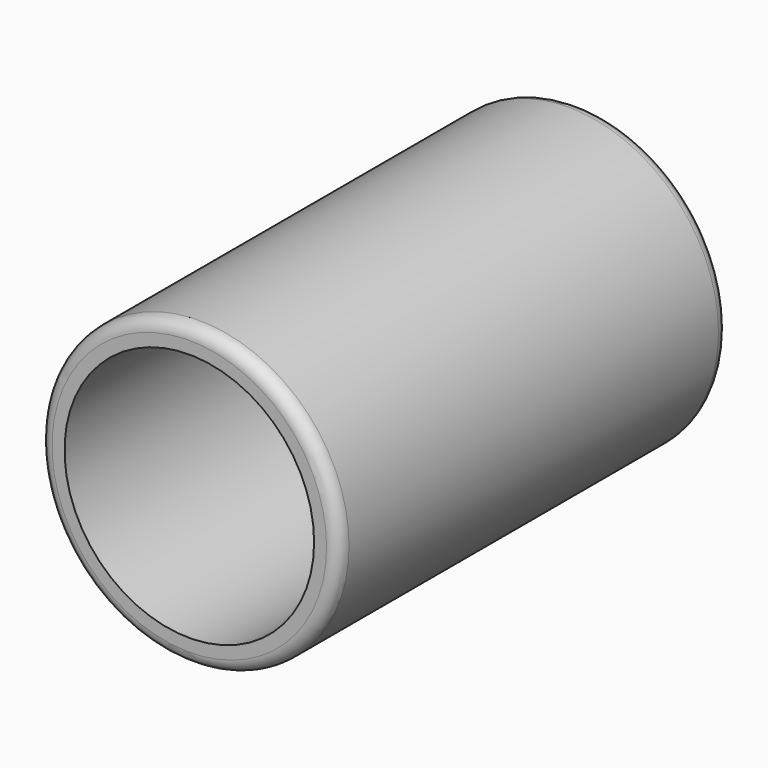
from build123d import *

# Parameters (mm, degrees)
F0_R     = 38.1
F0_R_2   = 31.75
F1_DEPTH = 123.825
F2_R     = 3.175
F3_R     = 3.17499
F4_DEPTH = 9.525


# Not quite as in the source:
# - a fillet or chamfer is up to 0.001 mm smaller than in the source, because OpenCascade refuses the exact size


with BuildPart() as f1:
    # F0 (on Front) → F1 (new body)
    with BuildSketch(Plane.XZ):
        Circle(F0_R)
        Circle(F0_R_2, mode=Mode.SUBTRACT)
    extrude(amount=F1_DEPTH)

    # F2
    f2_edges = [f1.edges().sort_by_distance(p)[0] for p in [
        (-38.1, -123.825, 0),
    ]]
    fillet(f2_edges, radius=F2_R)

    # F3 (radius 3.175 in the source; OpenCascade refuses exactly that, so slightly less here)
    f3_edges = [f1.edges().sort_by_distance(p)[0] for p in [
        (-38.1, 0, 0),
        (-31.75, 0, 0),
    ]]
    fillet(f3_edges, radius=F3_R)


with BuildPart() as f4:
    # F0 (on Front) → F4 (new body)
    with BuildSketch(Plane.XZ):
        Circle(F0_R_2)
    extrude(amount=F4_DEPTH)


solid = Compound([f1.part, f4.part])
